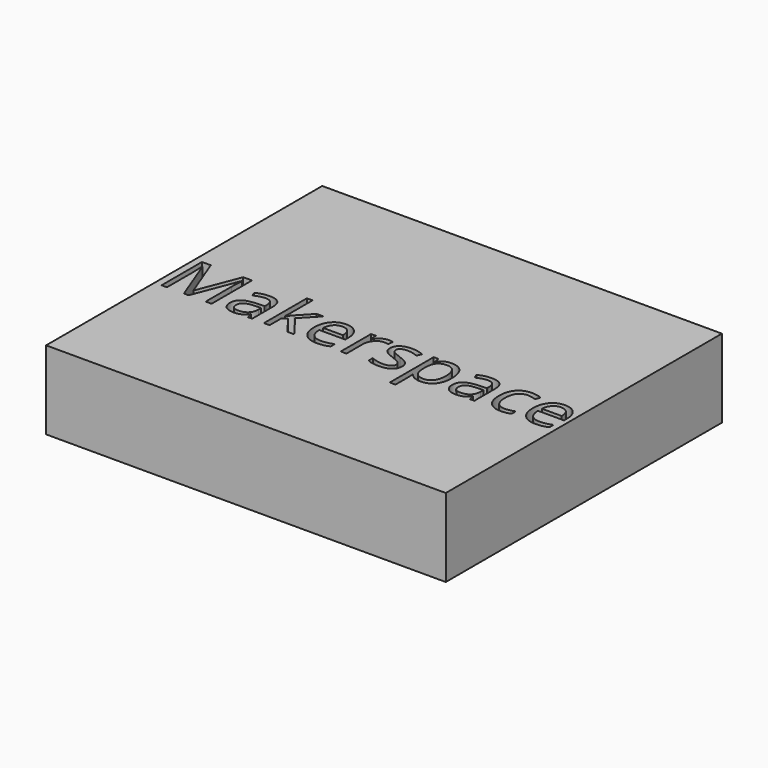
from build123d import *

# Parameters (mm, degrees)
F0_W         = 129.5075677335
F0_H         = 111.8361763656
F1_DEPTH     = 25.4
F2_TEXT_SIZE = 22.9267656975
F3_DEPTH     = 25.4


# Not quite as in the source:
# - Text() gives the source's letters only with a copy of the font that has no kerning and outlines rounded to 1/6400 em; it was checked with that copy


with BuildPart() as f1:
    # F0 (on Top) → F1 (new body)
    with BuildSketch(Plane.XY):
        with Locations((7.4979607016, 5.3585302085)):
            Rectangle(F0_W, F0_H)
    extrude(amount=F1_DEPTH)

    # F2 (on face) → F3 (cut)
    with BuildSketch(Plane.XY.offset(25.4)):
        with Locations((-57.2558231652, -6.6156715146)):
            Text('Makerspace', F2_TEXT_SIZE, font='Open Sans', text_align=(TextAlign.LEFT, TextAlign.BOTTOM))
    extrude(amount=-F3_DEPTH, mode=Mode.SUBTRACT)


solid = f1.part
